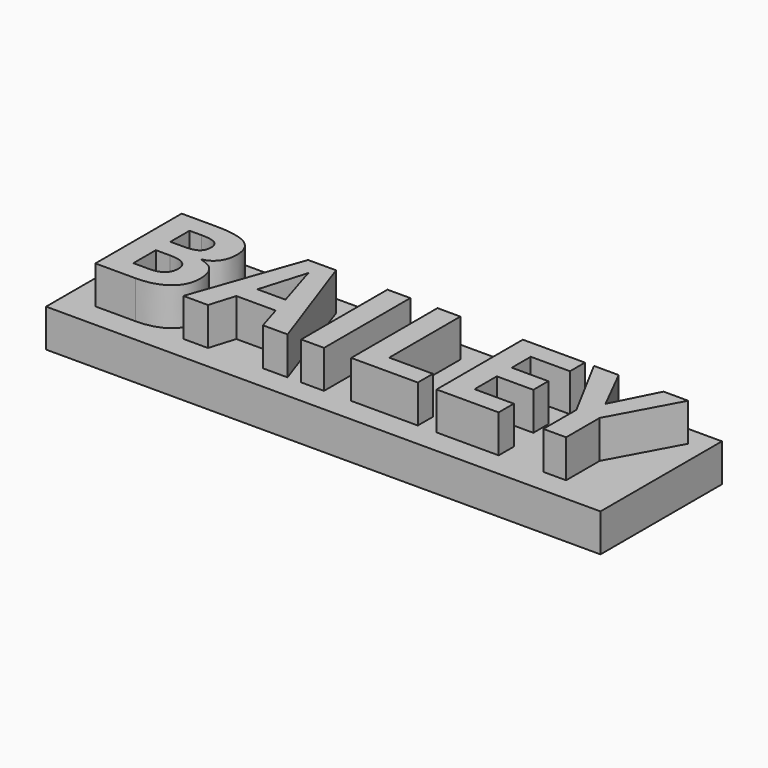
from build123d import *

# Parameters (mm, degrees)
F0_TEXT_SIZE = 25.3502049546
F1_DEPTH     = 12.7
F2_W         = 93.0067040026
F2_H         = 25.4712393507
F3_DEPTH     = 6.35


# Not quite as in the source:
# - Text() gives the source's letters only with a copy of the font that has no kerning and outlines rounded to 1/6400 em; it was checked with that copy


with BuildPart() as f1:
    # F0 (on Top) → F1 (new body)
    with BuildSketch(Plane.XY):
        with Locations((-44.9848153081, -9.6356201008)):
            Text('BAILEY', F0_TEXT_SIZE, font='Open Sans', font_style=FontStyle.BOLD, text_align=(TextAlign.LEFT, TextAlign.BOTTOM))
    extrude(amount=F1_DEPTH)


with BuildPart() as f3:
    # F2 (on Top) → F3 (new body)
    with BuildSketch(Plane.XY):
        with Locations((-1.2076664716, -0.9820680134)):
            Rectangle(F2_W, F2_H)
    extrude(amount=F3_DEPTH)


solid = Compound([f1.part, f3.part])
